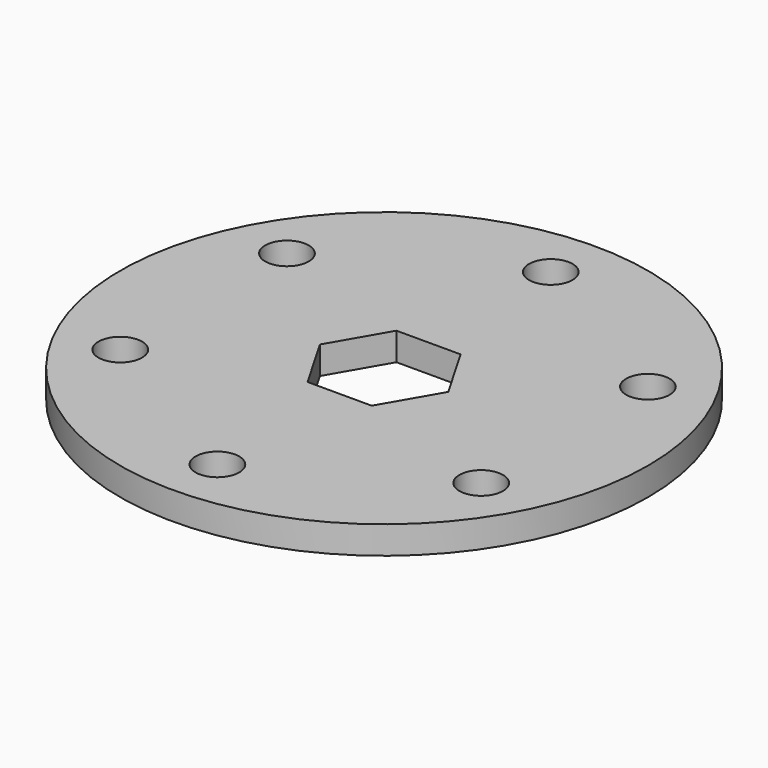
from build123d import *

# Parameters (mm, degrees)
F0_R            = 30.1625
F1_DEPTH        = 3.175
F2_R            = 2.4892
F3_DEPTH        = 3.176
F3_COPIES_COUNT = 6
F4_R            = 2.3622
F5_DEPTH        = 3.176


# Not quite as in the source:
# - a pattern or mirror of a feature is missing from the dataset's text; its kind, count and spacing are read off the source's solid


with BuildPart() as f1:
    # F0 (on Top) → F1 (new body)
    with BuildSketch(Plane.XY):
        Circle(F0_R)
        Polygon((7.3323484187, 0), (3.6661742094, -6.35), (-3.6661742094, -6.35), (-7.3323484187, 0), (-3.6661742094, 6.35), (3.6661742094, 6.35), align=None, mode=Mode.SUBTRACT)
    extrude(amount=F1_DEPTH)

    # F2 (on face) → F3 (cut, through all)
    with BuildSketch(Plane.XY.offset(3.175)):
        with Locations((0, 23.8125)):
            Circle(F2_R)
    f3 = extrude(amount=-F3_DEPTH, mode=Mode.SUBTRACT)

    # F3_copies: F3 ×6 about axis
    f3_copies_axis = Axis((0, 0, 0), (0, 0, 1))
    for i in range(1, F3_COPIES_COUNT):
        add(f3.rotate(f3_copies_axis, i * 360 / F3_COPIES_COUNT), mode=Mode.SUBTRACT)

    # F4 (on face) → F5 (cut, through all)
    with BuildSketch(Plane.XY.offset(3.175)):
        with Locations((0, 40.2743678674)):
            Circle(F4_R)
        with Locations((38.3032, 12.4454641087)):
            Circle(F4_R)
        with Locations((23.6726794779, -32.5826480425)):
            Circle(F4_R)
        with Locations((-23.6726794779, -32.5826480425)):
            Circle(F4_R)
        with Locations((-38.3032, 12.4454641087)):
            Circle(F4_R)
    extrude(amount=-F5_DEPTH, mode=Mode.SUBTRACT)


solid = f1.part
